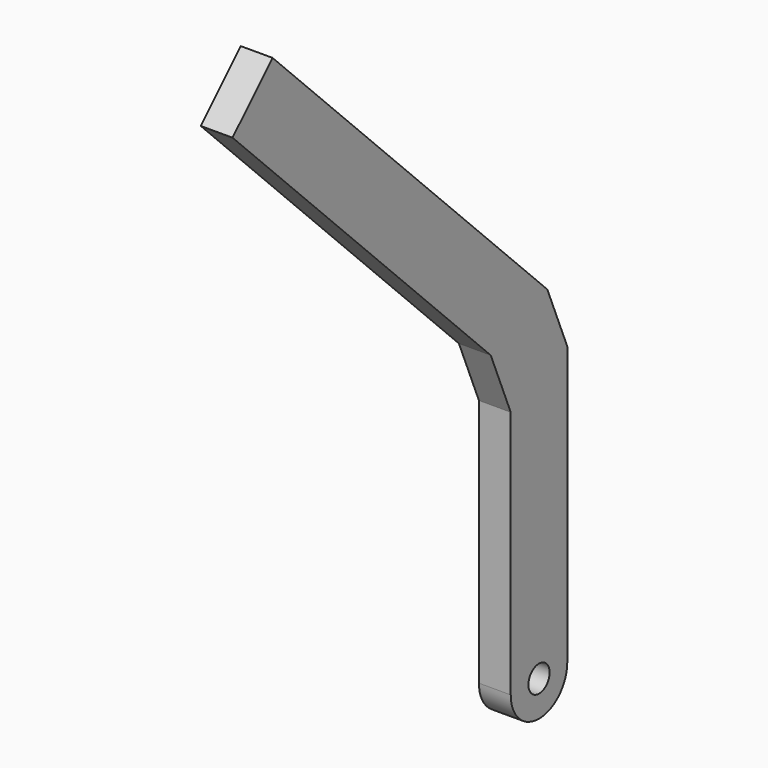
from build123d import *

# Parameters (mm, degrees)
F1_DEPTH = 2.8575
F3_D     = 4.7625
F4_R     = 6.34999
F5_SIZE  = 6.35


# Not quite as in the source:
# - a fillet or chamfer is up to 0.001 mm smaller than in the source, because OpenCascade refuses the exact size


with BuildPart() as f1:
    # F0 (on Right) → F1 (new body, symmetric)
    with BuildSketch(Plane.YZ):
        Polygon((6.35, -6.35), (6.35, 56.3145122421), (-59.8537438789, 122.5182561211), (-68.834, 113.538), (-6.35, 51.054), (-6.35, -6.35), align=None)
    extrude(amount=F1_DEPTH, both=True)

    # F3 (through all)
    with Locations(Plane.YZ.offset(2.8575)):
        with Locations((0, 0)):
            Hole(F3_D / 2)

    # F4 (radius 6.35 in the source; OpenCascade refuses exactly that, so slightly less here)
    f4_edges = [f1.edges().sort_by_distance(p)[0] for p in [
        (0, -6.35, -6.35),
        (0, 6.35, -6.35),
    ]]
    fillet(f4_edges, radius=F4_R)

    # F5
    f5_edges = [f1.edges().sort_by_distance(p)[0] for p in [
        (0, -6.35, 51.054),
        (0, 6.35, 56.314512),
    ]]
    chamfer(f5_edges, length=F5_SIZE)


solid = f1.part
